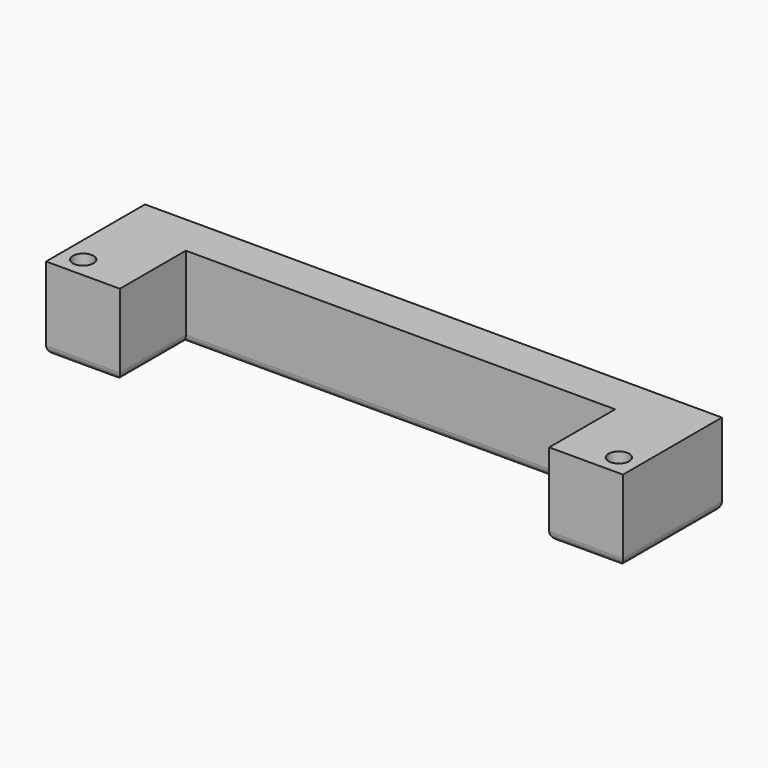
from build123d import *

# Parameters (mm, degrees)
F1_DEPTH     = 20
F3_D         = 5
F5_T1_DEPTH  = 150
F5_T3_DEPTH  = 40
F5_T5_DEPTH  = 27.906979831
F5_T7_DEPTH  = 25
F5_T9_DEPTH  = 104.186040338
F5_T11_DEPTH = 27.906979831
F5_T21_DEPTH = 30
F5_T25_DEPTH = 109.186040338
F5_T32_DEPTH = 109.186040338
F5_T36_DEPTH = 30


# Not quite as in the source:
# - a fillet or chamfer that OpenCascade refuses, or shapes differently, is made with other operations: its cross-section is extruded or revolved along the edge and cut away or added


with BuildPart() as f1:
    # F0 (on Top) → F1 (new body)
    with BuildSketch(Plane.XY):
        Polygon((70, 30), (0, 30), (0, 20), (52.093020169, 20), (52.093020169, 0), (70, 0), align=None)
    extrude(amount=F1_DEPTH)

    # F3 (through all)
    with Locations(Plane.XY.offset(20)):
        with Locations((65, 5)):
            Hole(F3_D / 2)

    # F4: F1 across face


with BuildPart() as f1_1:
    add(f1.part)
    add(f1.part.mirror(Plane(origin=(0, 25, 10), x_dir=(0, -1, 0), z_dir=(-1, 0, 0))))

    # F5: fillet of radius 2 on 10 edges, made by hand

    # F5_s2 → F5_t1 (cut)
    with BuildSketch(Plane.YZ.offset(-75)):
        with BuildLine():
            ThreePointArc((30, 2), (29.4142135624, 0.5857864376), (28, 0))
            Line((28, 0), (30, 0))
            Line((30, 0), (30, 2))
        make_face()
    extrude(amount=F5_T1_DEPTH, mode=Mode.SUBTRACT)

    # F5_s4 → F5_t3 (cut)
    with BuildSketch(Plane.XZ.offset(-35)):
        with BuildLine():
            ThreePointArc((-68, 0), (-69.4142135624, 0.5857864376), (-70, 2))
            Line((-70, 2), (-70, 0))
            Line((-70, 0), (-68, 0))
        make_face()
        with BuildLine():
            ThreePointArc((68, 0), (69.4142135624, 0.5857864376), (70, 2))
            Line((70, 2), (70, 0))
            Line((70, 0), (68, 0))
        make_face()
    extrude(amount=F5_T3_DEPTH, mode=Mode.SUBTRACT)

    # F5_s6 → F5_t5 (cut)
    with BuildSketch(Plane.YZ.offset(-75)):
        with BuildLine():
            ThreePointArc((2, 0), (0.5857864376, 0.5857864376), (0, 2))
            Line((0, 2), (0, 0))
            Line((0, 0), (2, 0))
        make_face()
    extrude(amount=F5_T5_DEPTH, mode=Mode.SUBTRACT)

    # F5_s8 → F5_t7 (cut)
    with BuildSketch(Plane.XZ.offset(-20)):
        with BuildLine():
            ThreePointArc((-54.093020169, 0), (-52.6788066067, 0.5857864376), (-52.093020169, 2))
            Line((-52.093020169, 2), (-52.093020169, 0))
            Line((-52.093020169, 0), (-54.093020169, 0))
        make_face()
        with BuildLine():
            ThreePointArc((54.093020169, 0), (52.6788066067, 0.5857864376), (52.093020169, 2))
            Line((52.093020169, 2), (52.093020169, 0))
            Line((52.093020169, 0), (54.093020169, 0))
        make_face()
    extrude(amount=F5_T7_DEPTH, mode=Mode.SUBTRACT)

    # F5_s10 → F5_t9 (cut)
    with BuildSketch(Plane.YZ.offset(-52.093020169)):
        with BuildLine():
            ThreePointArc((22, 0), (20.5857864376, 0.5857864376), (20, 2))
            Line((20, 2), (20, 0))
            Line((20, 0), (22, 0))
        make_face()
    extrude(amount=F5_T9_DEPTH, mode=Mode.SUBTRACT)

    # F5_s12 → F5_t11 (cut)
    with BuildSketch(Plane.YZ.offset(47.093020169)):
        with BuildLine():
            ThreePointArc((2, 0), (0.5857864376, 0.5857864376), (0, 2))
            Line((0, 2), (0, 0))
            Line((0, 0), (2, 0))
        make_face()
    extrude(amount=F5_T11_DEPTH, mode=Mode.SUBTRACT)

    # F5_s13 → F5_t14 (revolve, cut)
    with BuildSketch(Plane.XZ.offset(-5)):
        with BuildLine():
            ThreePointArc((69.5, 0), (68.0857864376, 0.5857864376), (67.5, 2))
            Line((67.5, 2), (67.5, 0))
            Line((67.5, 0), (69.5, 0))
        make_face()
    revolve(axis=Axis((65, 5, 0), (0, 0, 1)), mode=Mode.SUBTRACT)

    # F5_s15 → F5_t16 (revolve, cut)
    with BuildSketch(Plane.XZ.offset(-5)):
        with BuildLine():
            ThreePointArc((-69.5, 0), (-68.0857864376, 0.5857864376), (-67.5, 2))
            Line((-67.5, 2), (-67.5, 0))
            Line((-67.5, 0), (-69.5, 0))
        make_face()
    revolve(axis=Axis((-65, 5, 0), (0, 0, -1)), mode=Mode.SUBTRACT)


with BuildPart() as f5_tool19:
    # F5_s20 → F5_t21 (new body)
    with BuildSketch(Plane.XZ.offset(-25)):
        with BuildLine():
            ThreePointArc((-54.093020169, 0), (-52.6788066067, 0.5857864376), (-52.093020169, 2))
            Line((-52.093020169, 2), (-52.093020169, 0))
            Line((-52.093020169, 0), (-54.093020169, 0))
        make_face()
    extrude(amount=F5_T21_DEPTH)

    split(bisect_by=Plane.XZ.offset(-20), keep=Keep.BOTTOM)


with BuildPart() as f5_tool23:
    # F5_s24 → F5_t25 (new body)
    with BuildSketch(Plane.YZ.offset(52.093020169)):
        with BuildLine():
            ThreePointArc((22, 0), (20.5857864376, 0.5857864376), (20, 2))
            Line((20, 2), (20, 0))
            Line((20, 0), (22, 0))
        make_face()
    extrude(amount=-F5_T25_DEPTH)

    split(bisect_by=Plane.YZ.offset(-52.093020169), keep=Keep.BOTTOM)


with BuildPart() as f5_tool19_1:
    add(f5_tool19.part)

    # F5_t27: intersect F5_tool23
    add(f5_tool23.part, mode=Mode.INTERSECT)


with BuildPart() as f1_2:
    add(f1_1.part)

    # F5_t17: cut F5_tool19
    add(f5_tool19_1.part, mode=Mode.SUBTRACT)


with BuildPart() as f5_tool30:
    # F5_s31 → F5_t32 (new body)
    with BuildSketch(Plane.YZ.offset(57.093020169)):
        with BuildLine():
            ThreePointArc((22, 0), (20.5857864376, 0.5857864376), (20, 2))
            Line((20, 2), (20, 0))
            Line((20, 0), (22, 0))
        make_face()
    extrude(amount=-F5_T32_DEPTH)

    split(bisect_by=Plane.YZ.offset(52.093020169), keep=Keep.TOP)


with BuildPart() as f5_tool34:
    # F5_s35 → F5_t36 (new body)
    with BuildSketch(Plane.XZ.offset(-25)):
        with BuildLine():
            ThreePointArc((54.093020169, 0), (52.6788066067, 0.5857864376), (52.093020169, 2))
            Line((52.093020169, 2), (52.093020169, 0))
            Line((52.093020169, 0), (54.093020169, 0))
        make_face()
    extrude(amount=F5_T36_DEPTH)

    split(bisect_by=Plane.XZ.offset(-20), keep=Keep.BOTTOM)


with BuildPart() as f5_tool30_1:
    add(f5_tool30.part)

    # F5_t38: intersect F5_tool34
    add(f5_tool34.part, mode=Mode.INTERSECT)


with BuildPart() as f1_3:
    add(f1_2.part)

    # F5_t28: cut F5_tool30
    add(f5_tool30_1.part, mode=Mode.SUBTRACT)


solid = f1_3.part
